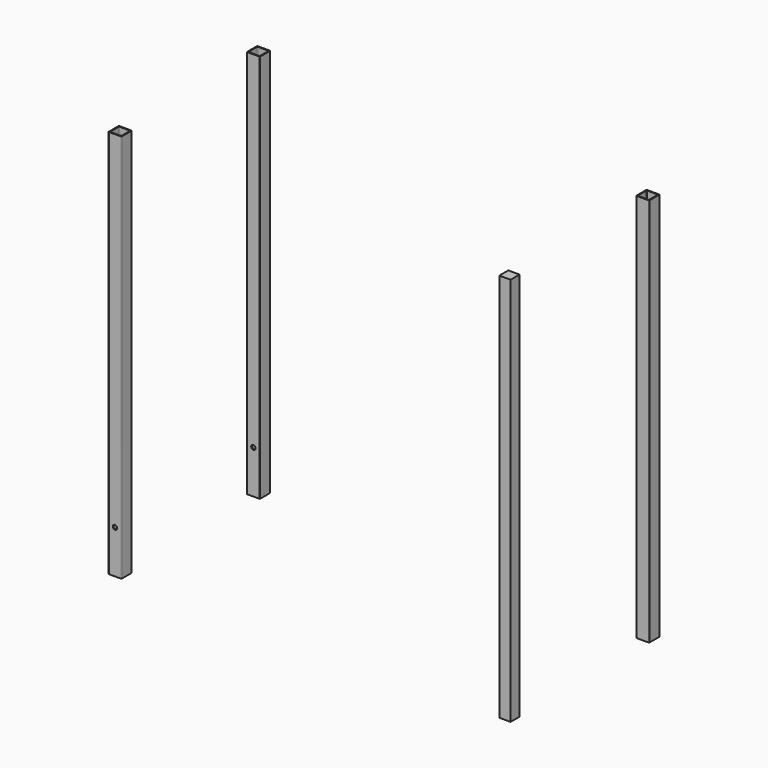
from build123d import *

# Parameters (mm, degrees)
F2_DEPTH = 900
F3_R     = 5
F4_DEPTH = 30
F5_R     = 5
F6_DEPTH = 30
F7_DEPTH = 25


with BuildPart() as f2:
    # F0 (on Top) → F2 (new body)
    with BuildSketch(Plane.XY):
        with BuildLine():
            ThreePointArc((0, 1), (0.2928932188, 0.2928932188), (1, 0))
            Line((1, 0), (29, 0))
            ThreePointArc((29, 0), (29.7071067812, 0.2928932188), (30, 1))
            Line((30, 1), (30, 29))
            ThreePointArc((30, 29), (29.7071067812, 29.7071067812), (29, 30))
            Line((29, 30), (1, 30))
            ThreePointArc((1, 30), (0.2928932188, 29.7071067812), (0, 29))
            Line((0, 29), (0, 1))
        make_face()
        with BuildLine():
            Line((3, 28), (27, 28))
            ThreePointArc((27, 28), (27.7071067812, 27.7071067812), (28, 27))
            Line((28, 27), (28, 2))
            Line((28, 2), (3, 2))
            ThreePointArc((3, 2), (2.2928932188, 2.2928932188), (2, 3))
            Line((2, 3), (2, 27))
            ThreePointArc((2, 27), (2.2928932188, 27.7071067812), (3, 28))
        make_face(mode=Mode.SUBTRACT)
    extrude(amount=F2_DEPTH)

    # F3 (on face) → F4 (cut)
    with BuildSketch(Plane.XZ):
        with Locations((15, 100)):
            Circle(F3_R)
    extrude(amount=-F4_DEPTH, mode=Mode.SUBTRACT)

    # F0 (on Top) → F7 (cut)
    with BuildSketch(Plane.XY):
        with BuildLine():
            ThreePointArc((28, 27), (27.7071067812, 27.7071067812), (27, 28))
            Line((27, 28), (3, 28))
            ThreePointArc((3, 28), (2.2928932188, 27.7071067812), (2, 27))
            Line((2, 27), (2, 3))
            ThreePointArc((2, 3), (2.2928932188, 2.2928932188), (3, 2))
            Line((3, 2), (28, 2))
            Line((28, 2), (28, 27))
        make_face()
    extrude(amount=-F7_DEPTH, mode=Mode.SUBTRACT)


with BuildPart() as f2b:
    # F0 (on Top) → F2, piece 2 (new body)
    with BuildSketch(Plane.XY):
        with BuildLine():
            ThreePointArc((29, 400), (29.7071067812, 400.2928932188), (30, 401))
            Line((30, 401), (30, 429))
            ThreePointArc((30, 429), (29.7071067812, 429.7071067812), (29, 430))
            Line((29, 430), (1, 430))
            ThreePointArc((1, 430), (0.2928932188, 429.7071067812), (0, 429))
            Line((0, 429), (0, 401))
            ThreePointArc((0, 401), (0.2928932188, 400.2928932188), (1, 400))
            Line((1, 400), (29, 400))
        make_face()
        with BuildLine():
            Line((3, 428), (27, 428))
            ThreePointArc((27, 428), (27.7071067812, 427.7071067812), (28, 427))
            Line((28, 427), (28, 402))
            Line((28, 402), (3, 402))
            ThreePointArc((3, 402), (2.2928932188, 402.2928932188), (2, 403))
            Line((2, 403), (2, 427))
            ThreePointArc((2, 427), (2.2928932188, 427.7071067812), (3, 428))
        make_face(mode=Mode.SUBTRACT)
    extrude(amount=F2_DEPTH)

    # F5 (on face) → F6 (cut)
    with BuildSketch(Plane(origin=(0, 430, 0), x_dir=(-1, 0, 0), z_dir=(0, 1, 0))):
        with Locations((-15, 100)):
            Circle(F5_R)
    extrude(amount=-F6_DEPTH, mode=Mode.SUBTRACT)


with BuildPart() as f2c:
    # F0 (on Top) → F2, piece 3 (new body)
    with BuildSketch(Plane.XY):
        with BuildLine():
            ThreePointArc((928, 27), (927.7071067812, 27.7071067812), (927, 28))
            Line((927, 28), (903, 28))
            ThreePointArc((903, 28), (902.2928932188, 27.7071067812), (902, 27))
            Line((902, 27), (902, 3))
            ThreePointArc((902, 3), (902.2928932188, 2.2928932188), (903, 2))
            Line((903, 2), (928, 2))
            Line((928, 2), (928, 27))
        make_face()
    extrude(amount=F2_DEPTH)


with BuildPart() as f2d:
    # F0 (on Top) → F2, piece 4 (new body)
    with BuildSketch(Plane.XY):
        with BuildLine():
            ThreePointArc((929, 400), (929.7071067812, 400.2928932188), (930, 401))
            Line((930, 401), (930, 429))
            ThreePointArc((930, 429), (929.7071067812, 429.7071067812), (929, 430))
            Line((929, 430), (901, 430))
            ThreePointArc((901, 430), (900.2928932188, 429.7071067812), (900, 429))
            Line((900, 429), (900, 401))
            ThreePointArc((900, 401), (900.2928932188, 400.2928932188), (901, 400))
            Line((901, 400), (929, 400))
        make_face()
        with BuildLine():
            Line((903, 428), (927, 428))
            ThreePointArc((927, 428), (927.7071067812, 427.7071067812), (928, 427))
            Line((928, 427), (928, 402))
            Line((928, 402), (903, 402))
            ThreePointArc((903, 402), (902.2928932188, 402.2928932188), (902, 403))
            Line((902, 403), (902, 427))
            ThreePointArc((902, 427), (902.2928932188, 427.7071067812), (903, 428))
        make_face(mode=Mode.SUBTRACT)
    extrude(amount=F2_DEPTH)


solid = Compound([f2.part, f2b.part, f2c.part, f2d.part])
